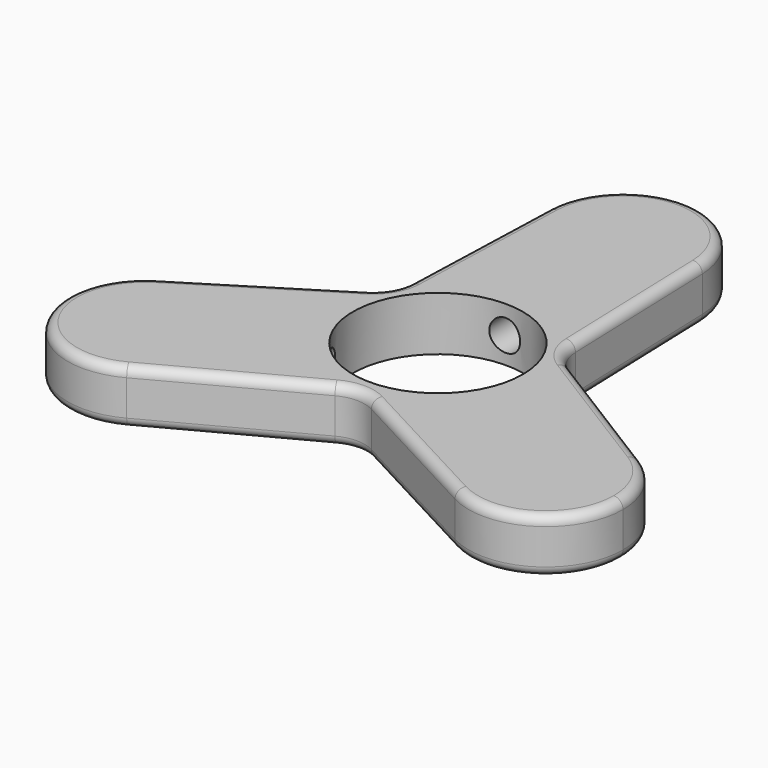
from build123d import *

# Parameters (mm, degrees)
F0_R      = 11
F1_DEPTH  = 7
F3_R      = 8.5
F4_DEPTH  = 4.2
F6_R      = 2
F7_DEPTH  = 12
F9_R      = 2
F10_DEPTH = 12
F12_R     = 2
F13_DEPTH = 12
F14_R     = 1.2


# Not quite as in the source:
# - a feature names something its author has since deleted; it is built from what else it names


with BuildPart() as f1:
    # F0 (on Top) → F1 (new body)
    with BuildSketch(Plane.XY):
        with BuildLine():
            ThreePointArc((9.9944429004, 30.3333333333), (9.9986106286, 30.1666898261), (10, 30))
            ThreePointArc((10, 30), (-0.1666898261, 20.0013893714), (-9.9944429004, 30.3333333333))
            Line((-9.9944429004, 30.3333333333), (-10.7092358725, 8.9014606966))
            ThreePointArc((-10.7092358725, 8.9014606966), (-11.3763303038, 6.5681273633), (-13.0635090303, 4.8237399724))
            Line((-13.0635090303, 4.8237399724), (-31.2666586983, -6.5112252183))
            ThreePointArc((-31.2666586983, -6.5112252183), (-21.1258144232, -6.2576042801), (-15.9807621135, -15))
            ThreePointArc((-15.9807621135, -15), (-17.4050562197, -20.1436629382), (-21.2722157979, -23.8221081151))
            Line((-21.2722157979, -23.8221081151), (-2.3542731578, -13.725200669))
            ThreePointArc((-2.3542731578, -13.725200669), (0, -13.1362547266), (2.3542731578, -13.725200669))
            Line((2.3542731578, -13.725200669), (21.2722157979, -23.8221081151))
            ThreePointArc((21.2722157979, -23.8221081151), (17.3205080757, -10), (31.2666586983, -6.5112252183))
            Line((31.2666586983, -6.5112252183), (13.0635090303, 4.8237399724))
            ThreePointArc((13.0635090303, 4.8237399724), (11.3763303038, 6.5681273633), (10.7092358725, 8.9014606966))
            Line((10.7092358725, 8.9014606966), (9.9944429004, 30.3333333333))
        make_face()
        Circle(F0_R, mode=Mode.SUBTRACT)
        with BuildLine():
            ThreePointArc((-9.9944429004, 30.3333333333), (-0.1666898261, 20.0013893714), (10, 30))
            ThreePointArc((10, 30), (9.9986106286, 30.1666898261), (9.9944429004, 30.3333333333))
            ThreePointArc((9.9944429004, 30.3333333333), (0, 40), (-9.9944429004, 30.3333333333))
        make_face()
        with BuildLine():
            ThreePointArc((-15.9807621135, -15), (-21.1258144232, -6.2576042801), (-31.2666586983, -6.5112252183))
            ThreePointArc((-31.2666586983, -6.5112252183), (-34.6410161514, -20), (-21.2722157979, -23.8221081151))
            ThreePointArc((-21.2722157979, -23.8221081151), (-17.4050562197, -20.1436629382), (-15.9807621135, -15))
        make_face()
        with BuildLine():
            ThreePointArc((35.9807621135, -15), (34.7231578335, -10.1450523096), (31.2666586983, -6.5112252183))
            ThreePointArc((31.2666586983, -6.5112252183), (17.3205080757, -10), (21.2722157979, -23.8221081151))
            ThreePointArc((21.2722157979, -23.8221081151), (31.1244250518, -23.5757058939), (35.9807621135, -15))
        make_face()
    extrude(amount=F1_DEPTH)

    # F3 (on offset) → F4 (cut)
    with BuildSketch(Plane.XY.offset(1.4)):
        with Locations((25.9807621135, -15)):
            Circle(F3_R)
        with Locations((-25.9807621135, -15)):
            Circle(F3_R)
        with Locations((0, 30)):
            Circle(F3_R)
    extrude(amount=F4_DEPTH, mode=Mode.SUBTRACT)

    # F6 (on offset) → F7 (cut)
    with BuildSketch(Plane.XZ.offset(-10)):
        with Locations((0, 3.4)):
            Circle(F6_R)
    extrude(amount=-F7_DEPTH, mode=Mode.SUBTRACT)

    # F9 (on line) → F10 (cut)
    with BuildSketch(Plane(origin=(8.8814954724, -5.1277338018, 0), x_dir=(0.5, 0.8660254038, 0), z_dir=(0.8660254038, -0.5, 0))):
        with Locations((0, 3.4)):
            Circle(F9_R)
    extrude(amount=F10_DEPTH, mode=Mode.SUBTRACT)

    # F12 (on line) → F13 (cut)
    with BuildSketch(Plane(origin=(-8.8814954724, -5.1277338018, 0), x_dir=(-0.5, 0.8660254038, 0), z_dir=(0.8660254038, 0.5, 0))):
        with Locations((0, 3.4)):
            Circle(F12_R)
    extrude(amount=-F13_DEPTH, mode=Mode.SUBTRACT)

    # F14
    f14_edges = [f1.edges().sort_by_distance(p)[0] for p in [
        (0, 40, 7),
        (0, 40, 0),
    ]]
    fillet(f14_edges, radius=F14_R)


solid = f1.part
